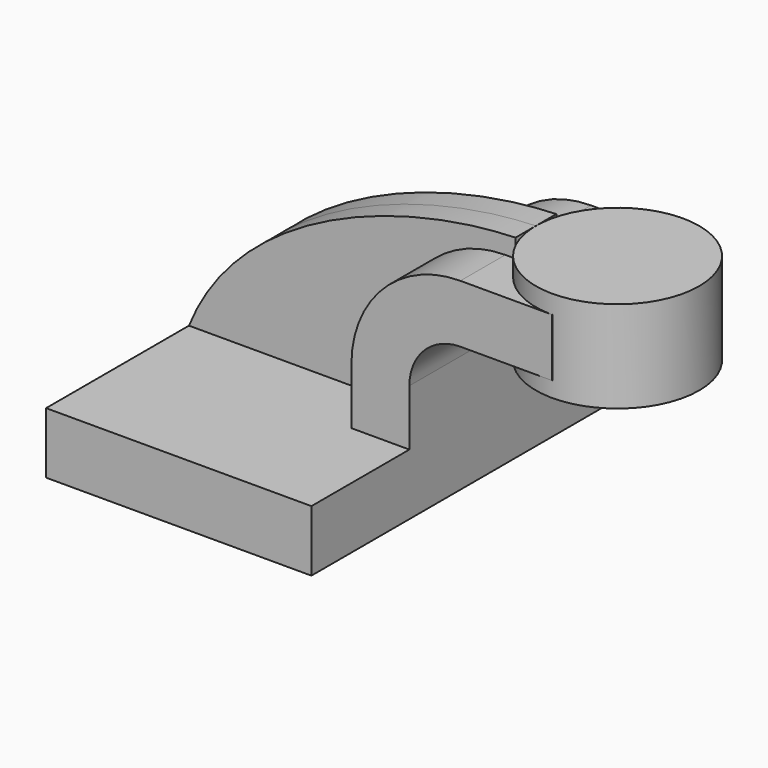
from build123d import *

# Parameters (mm, degrees)
F1_DEPTH = 63.5
F3_DEPTH = 25.4
F4_DEPTH = 7.9375


# Not quite as in the source:
# - a feature names something its author has since deleted; it is built from what else it names


with BuildPart() as f1:
    # F0 (on Front) → F1 (new body, symmetric)
    with BuildSketch(Plane.XZ):
        Polygon((-41.275, -9.525), (41.275, -9.525), (41.275, 9.525), (23.2382267714, 9.525), (-41.275, 9.525), align=None)
    extrude(amount=F1_DEPTH, both=True)

    # F0 (on Front) → F3 (join, symmetric)
    with BuildSketch(Plane.XZ):
        with BuildLine():
            Line((23.2382267714, 9.525), (41.275, 9.525))
            Line((41.275, 9.525), (41.275, 27.0002))
            ThreePointArc((41.275, 27.0002), (45.9246798487, 38.2255201513), (57.15, 42.8752))
            Line((57.15, 42.8752), (60.325, 42.8752))
            Line((60.325, 42.8752), (85.725, 42.8752))
            Line((85.725, 42.8752), (85.725, 60.9119732286))
            Line((85.725, 60.9119732286), (60.325, 60.9119732286))
            Line((60.325, 60.9119732286), (57.15, 60.9119732286))
            ThreePointArc((57.15, 60.9119732286), (33.170755188, 50.979444812), (23.2382267714, 27.0002))
            Line((23.2382267714, 27.0002), (23.2382267714, 9.525))
        make_face()
    extrude(amount=F3_DEPTH, both=True)

    # F0 (on Front) → F4 (join, symmetric)
    with BuildSketch(Plane.XZ):
        with BuildLine():
            add(Edge.make_bspline(
                [(-41.275, 9.525), (-25.8415896149, 48.0881909513), (23.9874106138, 65.5300151641), (60.325, 66.675)],
                knots=[0, 0, 0, 0, 116.5705044169, 116.5705044169, 116.5705044169, 116.5705044169], degree=3))
            Line((-41.275, 9.525), (23.2382267714, 9.525))
            Line((23.2382267714, 9.525), (23.2382267714, 27.0002))
            ThreePointArc((23.2382267714, 27.0002), (33.170755188, 50.979444812), (57.15, 60.9119732286))
            Line((57.15, 60.9119732286), (60.325, 60.9119732286))
            Line((60.325, 60.9119732286), (60.325, 66.675))
        make_face()
    extrude(amount=F4_DEPTH, both=True)


with BuildPart() as f5:
    # F0 (on Front) → F5 (revolve)
    with BuildSketch(Plane.XZ):
        Polygon((111.125, 66.675), (85.725, 66.675), (85.725, 60.9119732286), (85.725, 42.8752), (85.725, 38.1), (111.125, 38.1), align=None)
    revolve(axis=Axis((85.725, 0, 52.3875), (0, 0, -1)))


solid = Compound([f1.part, f5.part])
